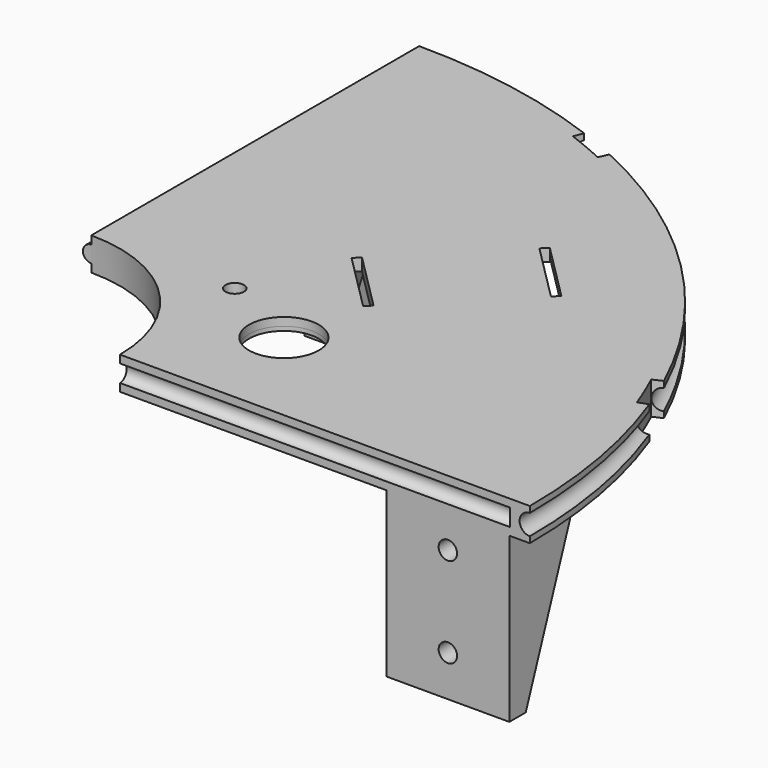
from build123d import *

# Parameters (mm, degrees)
F0_R      = 2.25
F1_DEPTH  = 8
F4_R      = 2.5
F6_W      = 30
F6_H      = 20
F6_W_2    = 20
F6_H_2    = 30
F7_DEPTH  = 40
F8_W      = 18
F8_H      = 15
F8_W_2    = 15
F8_H_2    = 18
F9_DEPTH  = 40
F10_SIZE2 = 39.99999
F10_SIZE  = 14.99999
F11_R     = 2.25
F12_DEPTH = 25
F13_SIZE2 = 14.99999
F13_SIZE  = 39.99999
F14_R     = 2.25
F15_DEPTH = 25
F17_DEPTH = 25
F19_DEPTH = 8.0010001
F22_R     = 2
F25_DEPTH = 48.001
F26_R     = 2.1
F28_R     = 8.5
F29_DEPTH = 8.0010001
F31_DEPTH = 6
F32_SIZE2 = 14.99999
F32_SIZE  = 45.99999
F33_SIZE2 = 14.99999
F33_SIZE  = 45.99999
F34_R     = 11
F34_R_2   = 8.5
F35_DEPTH = 1


# Not quite as in the source:
# - a fillet or chamfer is up to 0.001 mm smaller than in the source, because OpenCascade refuses the exact size


with BuildPart() as f1:
    # F0 (on Top) → F1 (new body)
    with BuildSketch(Plane.XY):
        with BuildLine():
            Line((35, 0), (135, 0))
            ThreePointArc((135, 0), (95.4594154602, 95.4594154602), (0, 135))
            Line((0, 135), (0, 35))
            ThreePointArc((0, 35), (24.7487373415, 24.7487373415), (35, 0))
        make_face()
        with Locations((35, 35)):
            Circle(F0_R, mode=Mode.SUBTRACT)
    extrude(amount=F1_DEPTH)

    # F5: sweep along a path in F3
    with BuildLine(Plane.XY.offset(4)) as f5_path:
        CenterArc((0, 0), 135, 0, 360)
    # F4 (on face) → F5 (sweep, cut)
    with BuildSketch(Plane.XZ):
        with Locations((135, 4)):
            Circle(F4_R)
    sweep(path=f5_path.line, mode=Mode.SUBTRACT)

    # F6 (on face) → F7 (join)
    with BuildSketch(Plane(origin=(0, 0, 0), x_dir=(1, 0, 0), z_dir=(0, 0, -1))):
        with Locations((115, -10)):
            Rectangle(F6_W, F6_H)
        with Locations((10, -115)):
            Rectangle(F6_W_2, F6_H_2)
    extrude(amount=F7_DEPTH)

    # F8 (on face) → F9 (cut)
    with BuildSketch(Plane(origin=(0, 0, -40), x_dir=(1, 0, 0), z_dir=(0, 0, -1))):
        with Locations((115, -12.5)):
            Rectangle(F8_W, F8_H)
        with Locations((12.5, -115)):
            Rectangle(F8_W_2, F8_H_2)
    extrude(amount=-F9_DEPTH, mode=Mode.SUBTRACT)

    # F10 (size 15 and 40 in the source; OpenCascade refuses exactly that, so slightly less here)
    f10_edges = [f1.edges().sort_by_distance(p)[0] for p in [
        (127, 20, -40),
    ]]
    f10_side = f1.faces().sort_by_distance((129.639445, 10, -40))[0]
    chamfer(f10_edges, length=F10_SIZE, length2=F10_SIZE2, reference=f10_side)

    # F11 (on face) → F12 (cut)
    with BuildSketch(Plane(origin=(0, 5, 0), x_dir=(-1, 0, 0), z_dir=(0, 1, 0))):
        with Locations((-115, -8)):
            Circle(F11_R)
        with Locations((-115, -30)):
            Circle(F11_R)
    extrude(amount=-F12_DEPTH, mode=Mode.SUBTRACT)

    # F13 (size 40 and 15 in the source; OpenCascade refuses exactly that, so slightly less here)
    f13_edges = [f1.edges().sort_by_distance(p)[0] for p in [
        (20, 127, -40),
    ]]
    chamfer(f13_edges, length=F13_SIZE, length2=F13_SIZE2)

    # F14 (on face) → F15 (cut)
    with BuildSketch(Plane.YZ.offset(5)):
        with Locations((115, -30)):
            Circle(F14_R)
        with Locations((115, -8)):
            Circle(F14_R)
    extrude(amount=-F15_DEPTH, mode=Mode.SUBTRACT)

    # F16 (on face) → F17 (cut)
    with BuildSketch(Plane.XY.offset(8)):
        with BuildLine():
            ThreePointArc((120.4496071259, 55.2099822787), (122.4117800348, 50.7110057948), (124.2059779255, 46.1424430169))
            Line((124.2059779255, 46.1424430169), (126.549486943, 47.0130551493))
            ThreePointArc((126.549486943, 47.0130551493), (124.7214362618, 51.6678172249), (122.7222412226, 56.2516800575))
            Line((122.7222412226, 56.2516800575), (120.4496071259, 55.2099822787))
        make_face()
        with BuildLine():
            Line((47.0017845491, 126.5536733928), (46.1313811315, 124.2100868484))
            ThreePointArc((46.1313811315, 124.2100868484), (50.7001036814, 122.416295838), (55.1992548973, 120.4545236128))
            Line((55.1992548973, 120.4545236128), (56.2407502727, 122.7272504734))
            ThreePointArc((56.2407502727, 122.7272504734), (51.6567094112, 124.7260372689), (47.0017845491, 126.5536733928))
        make_face()
    extrude(amount=-F17_DEPTH, mode=Mode.SUBTRACT)

    # F18 (on face) → F19 (cut, through all)
    with BuildSketch(Plane(origin=(0, 0, 0), x_dir=(1, 0, 0), z_dir=(0, 0, -1))):
        Polygon((44.5477272148, -58.6898628385), (45.9619407771, -60.1040764009), (60.1040764009, -45.9619407771), (58.6898628385, -44.5477272148), align=None)
        Polygon((84.1457069612, -70.0035713375), (70.0035713375, -84.1457069612), (71.4177848998, -85.5599205236), (85.5599205236, -71.4177848998), align=None)
    extrude(amount=-F19_DEPTH, mode=Mode.SUBTRACT)

    # F23: sweep along a path in F21
    with BuildLine(Plane(origin=(0, 0, 0), x_dir=(0, -1, 0), z_dir=(-1, 0, 0))) as f23_path:
        Line((-130, 4), (0, 4))
    # F22 (on Front) → F23 (sweep)
    with BuildSketch(Plane.XZ):
        with Locations((0, 4)):
            Circle(F22_R)
    sweep(path=f23_path.line)

    # F24 (on face) → F25 (cut, through all)
    with BuildSketch(Plane.XY.offset(8)):
        with BuildLine():
            ThreePointArc((0, 35), (-24.7487373415, -24.7487373415), (35, 0))
            ThreePointArc((35, 0), (24.7487373415, 24.7487373415), (0, 35))
        make_face()
    extrude(amount=-F25_DEPTH, mode=Mode.SUBTRACT)

    # F27: sweep along a path in F20
    with BuildLine(Plane.XZ) as f27_path:
        Line((0, 4), (130.2, 4))
    # F26 (on Right) → F27 (sweep, cut)
    with BuildSketch(Plane.YZ):
        with Locations((0, 4)):
            Circle(F26_R)
    sweep(path=f27_path.line, mode=Mode.SUBTRACT)

    # F28 (on face) → F29 (cut, through all)
    with BuildSketch(Plane(origin=(0, 0, 0), x_dir=(1, 0, 0), z_dir=(0, 0, -1))):
        with Locations((55, -25)):
            Circle(F28_R)
    extrude(amount=-F29_DEPTH, mode=Mode.SUBTRACT)

    # F30 (on face) → F31 (cut)
    with BuildSketch(Plane(origin=(0, 0, 0), x_dir=(1, 0, 0), z_dir=(0, 0, -1))):
        with BuildLine():
            Line((37, -40), (7, -40))
            ThreePointArc((7, -40), (5.5857864376, -40.5857864376), (5, -42))
            Line((5, -42), (5, -98))
            ThreePointArc((5, -98), (5.5857864376, -99.4142135624), (7, -100))
            Line((7, -100), (20, -100))
            Line((20, -100), (20, -106))
            Line((20, -106), (5, -106))
            Line((5, -106), (5, -124))
            Line((5, -124), (20, -124))
            ThreePointArc((20, -124), (88.8144132447, -88.8144132447), (124, -20))
            Line((124, -20), (124, -5))
            Line((124, -5), (106, -5))
            Line((106, -5), (106, -20))
            Line((106, -20), (100, -20))
            Line((100, -20), (100, -7))
            ThreePointArc((100, -7), (99.4142135624, -5.5857864376), (98, -5))
            Line((98, -5), (42, -5))
            ThreePointArc((42, -5), (40.5857864376, -5.5857864376), (40, -7))
            Line((40, -7), (40, -37))
            ThreePointArc((40, -37), (39.1213203436, -39.1213203436), (37, -40))
        make_face()
        with BuildLine():
            ThreePointArc((35.5519480519, -11.9293331629), (26.5165042945, -26.5165042945), (11.9293331629, -35.5519480519))
            ThreePointArc((11.9293331629, -35.5519480519), (11.2605211715, -36.6611645928), (12.2474487139, -37.5))
            Line((12.2474487139, -37.5), (29.7084973779, -37.5))
            ThreePointArc((29.7084973779, -37.5), (30.5062214131, -37.1030226892), (30.6705887637, -36.2272727273))
            ThreePointArc((30.6705887637, -36.2272727273), (31.8180194847, -31.8180194847), (36.2272727273, -30.6705887637))
            ThreePointArc((36.2272727273, -30.6705887637), (37.1030226892, -30.5062214131), (37.5, -29.7084973779))
            Line((37.5, -29.7084973779), (37.5, -12.2474487139))
            ThreePointArc((37.5, -12.2474487139), (36.6611645928, -11.2605211715), (35.5519480519, -11.9293331629))
        make_face()
    extrude(amount=-F31_DEPTH, mode=Mode.SUBTRACT)

    # F32 (size 46 and 15 in the source; OpenCascade refuses exactly that, so slightly less here)
    f32_edges = [f1.edges().sort_by_distance(p)[0] for p in [
        (20, 103, -40),
    ]]
    chamfer(f32_edges, length=F32_SIZE, length2=F32_SIZE2)

    # F33 (size 46 and 15 in the source; OpenCascade refuses exactly that, so slightly less here)
    f33_edges = [f1.edges().sort_by_distance(p)[0] for p in [
        (103, 20, -40),
    ]]
    f33_side = f1.faces().sort_by_distance((103, 20, -17))[0]
    chamfer(f33_edges, length=F33_SIZE, length2=F33_SIZE2, reference=f33_side)

    # F34 (on face) → F35 (join)
    with BuildSketch(Plane(origin=(0, 0, 6), x_dir=(1, 0, 0), z_dir=(0, 0, -1))):
        with BuildLine():
            Line((41.0121933088, -115.9655121146), (71.4177848998, -85.5599205236))
            Line((71.4177848998, -85.5599205236), (70.0035713375, -84.1457069612))
            Line((70.0035713375, -84.1457069612), (84.1457069612, -70.0035713375))
            Line((84.1457069612, -70.0035713375), (85.5599205236, -71.4177848998))
            Line((85.5599205236, -71.4177848998), (115.9655121146, -41.0121933088))
            ThreePointArc((115.9655121146, -41.0121933088), (116.5512985522, -39.5979797464), (115.9655121146, -38.1837661841))
            Line((115.9655121146, -38.1837661841), (91.9238815543, -14.1421356237))
            ThreePointArc((91.9238815543, -14.1421356237), (90.5096679919, -13.5563491861), (89.0954544295, -14.1421356237))
            Line((89.0954544295, -14.1421356237), (58.6898628385, -44.5477272148))
            Line((58.6898628385, -44.5477272148), (60.1040764009, -45.9619407771))
            Line((60.1040764009, -45.9619407771), (45.9619407771, -60.1040764009))
            Line((45.9619407771, -60.1040764009), (44.5477272148, -58.6898628385))
            Line((44.5477272148, -58.6898628385), (14.1421356237, -89.0954544295))
            ThreePointArc((14.1421356237, -89.0954544295), (13.5563491861, -90.5096679919), (14.1421356237, -91.9238815543))
            Line((14.1421356237, -91.9238815543), (38.1837661841, -115.9655121146))
            ThreePointArc((38.1837661841, -115.9655121146), (39.5979797464, -116.5512985522), (41.0121933088, -115.9655121146))
        make_face()
        with BuildLine():
            ThreePointArc((109.6015510839, -38.8908729653), (109.8944443027, -39.5979797464), (109.6015510839, -40.3050865276))
            Line((109.6015510839, -40.3050865276), (40.3050865276, -109.6015510839))
            ThreePointArc((40.3050865276, -109.6015510839), (39.5979797464, -109.8944443027), (38.8908729653, -109.6015510839))
            Line((38.8908729653, -109.6015510839), (37.4766594029, -108.1873375215))
            ThreePointArc((37.4766594029, -108.1873375215), (37.1837661841, -107.4802307404), (37.4766594029, -106.7731239592))
            Line((37.4766594029, -106.7731239592), (106.7731239592, -37.4766594029))
            ThreePointArc((106.7731239592, -37.4766594029), (107.4802307404, -37.1837661841), (108.1873375215, -37.4766594029))
            Line((108.1873375215, -37.4766594029), (109.6015510839, -38.8908729653))
        make_face(mode=Mode.SUBTRACT)
        with BuildLine():
            ThreePointArc((103.9446968344, -33.2340187158), (104.2375900532, -33.941125497), (103.9446968344, -34.6482322781))
            Line((103.9446968344, -34.6482322781), (34.6482322781, -103.9446968344))
            ThreePointArc((34.6482322781, -103.9446968344), (33.941125497, -104.2375900532), (33.2340187158, -103.9446968344))
            Line((33.2340187158, -103.9446968344), (31.8198051534, -102.530483272))
            ThreePointArc((31.8198051534, -102.530483272), (31.5269119346, -101.8233764909), (31.8198051534, -101.1162697097))
            Line((31.8198051534, -101.1162697097), (101.1162697097, -31.8198051534))
            ThreePointArc((101.1162697097, -31.8198051534), (101.8233764909, -31.5269119346), (102.530483272, -31.8198051534))
            Line((102.530483272, -31.8198051534), (103.9446968344, -33.2340187158))
        make_face(mode=Mode.SUBTRACT)
        with BuildLine():
            ThreePointArc((26.1629509039, -96.8736290226), (25.8700576851, -96.1665222414), (26.1629509039, -95.4594154602))
            Line((26.1629509039, -95.4594154602), (95.4594154602, -26.1629509039))
            ThreePointArc((95.4594154602, -26.1629509039), (96.1665222414, -25.8700576851), (96.8736290226, -26.1629509039))
            Line((96.8736290226, -26.1629509039), (98.2878425849, -27.5771644663))
            ThreePointArc((98.2878425849, -27.5771644663), (98.5807358037, -28.2842712475), (98.2878425849, -28.9913780286))
            Line((98.2878425849, -28.9913780286), (28.9913780286, -98.2878425849))
            ThreePointArc((28.9913780286, -98.2878425849), (28.2842712475, -98.5807358037), (27.5771644663, -98.2878425849))
            Line((27.5771644663, -98.2878425849), (26.1629509039, -96.8736290226))
        make_face(mode=Mode.SUBTRACT)
        with BuildLine():
            ThreePointArc((89.8025612107, -20.5060966544), (90.5096679919, -20.2132034356), (91.2167747731, -20.5060966544))
            Line((91.2167747731, -20.5060966544), (92.6309883354, -21.9203102168))
            ThreePointArc((92.6309883354, -21.9203102168), (92.9238815543, -22.627416998), (92.6309883354, -23.3345237792))
            Line((92.6309883354, -23.3345237792), (23.3345237792, -92.6309883354))
            ThreePointArc((23.3345237792, -92.6309883354), (22.627416998, -92.9238815543), (21.9203102168, -92.6309883354))
            Line((21.9203102168, -92.6309883354), (20.5060966544, -91.2167747731))
            ThreePointArc((20.5060966544, -91.2167747731), (20.2132034356, -90.5096679919), (20.5060966544, -89.8025612107))
            Line((20.5060966544, -89.8025612107), (89.8025612107, -20.5060966544))
        make_face(mode=Mode.SUBTRACT)
        with Locations((55, -25)):
            Circle(F34_R)
        with Locations((55, -25)):
            Circle(F34_R_2, mode=Mode.SUBTRACT)
    extrude(amount=F35_DEPTH)


solid = f1.part
